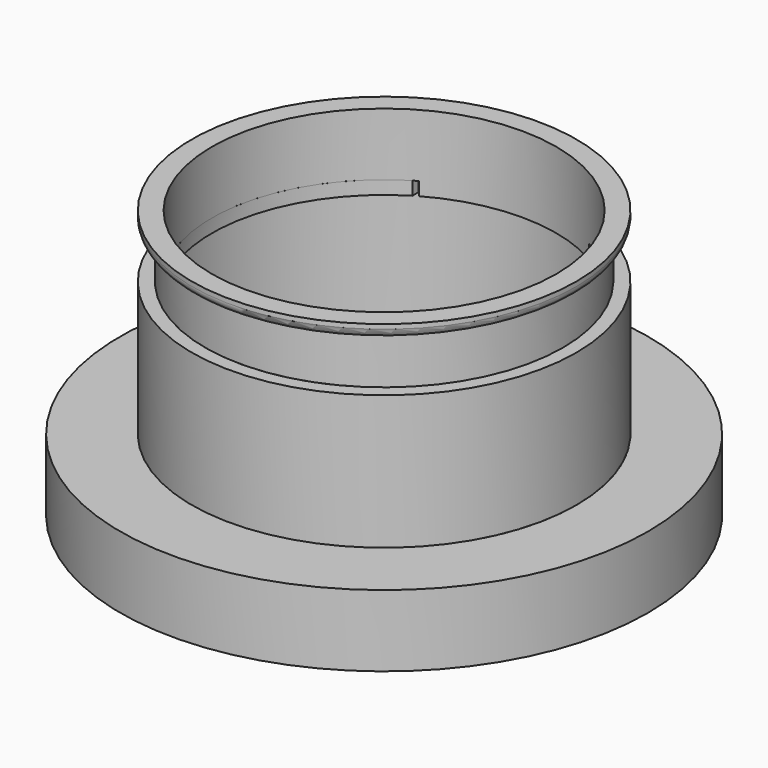
from build123d import *
from build123d import SkipClean  # not in build123d's __all__

# Parameters (mm, degrees)
F1_R      = 29.5
F2_DEPTH  = 8
F0_R      = 28
F3_DEPTH  = 6
F4_R      = 21.5
F5_DEPTH  = 15
F6_R      = 20.75
F7_DEPTH  = 21.5
F8_R      = 20
F9_DEPTH  = 7
F12_DEPTH = 1.5
F14_DEPTH = 2
F15_DEPTH = 1.5
F17_DEPTH = 2
F19_DEPTH = 2
F20_R     = 0.49999
F20_2_R   = 0.49999
F21_R     = 21.5
F22_DEPTH = 1.5
F10_R     = 19.25
F23_DEPTH = 50
F24_R     = 1


# Not quite as in the source:
# - a fillet or chamfer is up to 0.001 mm smaller than in the source, because OpenCascade refuses the exact size
# - a feature of the source that left no trace in its solid (it failed there, or was rolled back) is left out


with BuildPart() as f2:
    # F1 (on Top) → F2 (new body)
    with BuildSketch(Plane.XY):
        Circle(F1_R)
    extrude(amount=F2_DEPTH)

    # F0 (on Top) → F3 (cut)
    with BuildSketch(Plane.XY):
        Circle(F0_R)
    extrude(amount=F3_DEPTH, mode=Mode.SUBTRACT)


with BuildPart() as f5:
    # F4 (on face) → F5 (new body)
    with BuildSketch(Plane.XY.offset(8)):
        Circle(F4_R)
    extrude(amount=F5_DEPTH)


with BuildPart() as f7_tool:
    # F6 (on Top) → F7 (new body)
    with BuildSketch(Plane.XY):
        Circle(F6_R)
    extrude(amount=F7_DEPTH)


with BuildPart() as f2_1:
    add(f2.part, clean=False)

    # F7: cut by f7_tool
    add(f7_tool.part, mode=Mode.SUBTRACT)

    # F11 (on face) → F14 (cut)
    with BuildSketch(Plane(origin=(0, 0, 21.5), x_dir=(1, 0, 0), z_dir=(0, 0, -1))):
        with BuildLine():
            ThreePointArc((10, 17.3205080757), (0, 20), (-10, 17.3205080757))
            Line((-10, 17.3205080757), (-10, -17.3205080757))
            ThreePointArc((-10, -17.3205080757), (0, -20), (10, -17.3205080757))
            Line((10, -17.3205080757), (10, 17.3205080757))
        make_face()
    extrude(amount=F14_DEPTH, mode=Mode.SUBTRACT)

    # F16 (on face) → F17 (cut)
    with BuildSketch(Plane(origin=(0, 0, 6), x_dir=(1, 0, 0), z_dir=(0, 0, -1))):
        with BuildLine():
            Line((-18.1813778356, 10), (-19.0328663107, 10))
            ThreePointArc((-19.0328663107, 10), (-21.5, 0), (-19.0328663107, -10))
            Line((-19.0328663107, -10), (-18.1813778356, -10))
            ThreePointArc((-18.1813778356, -10), (-20.75, 0), (-18.1813778356, 10))
        make_face()
        with BuildLine():
            ThreePointArc((21.5, 0), (20.8741062764, 5.1499210829), (19.0328663107, 10))
            Line((19.0328663107, 10), (18.1813778356, 10))
            ThreePointArc((18.1813778356, 10), (20.0975880405, 5.1623110092), (20.75, 0))
            ThreePointArc((20.75, 0), (20.0975880405, -5.1623110092), (18.1813778356, -10))
            Line((18.1813778356, -10), (19.0328663107, -10))
            ThreePointArc((19.0328663107, -10), (20.8741062764, -5.1499210829), (21.5, 0))
        make_face()
    extrude(amount=-F17_DEPTH, mode=Mode.SUBTRACT)

    # F20 (radius 0.5 in the source; OpenCascade refuses exactly that, so slightly less here)
    f20_edges = [f2_1.edges().sort_by_distance(p)[0] for p in [
        (-28, 0, 0),
        (0, -20.75, 6),
        (0, 20.75, 6),
    ]]
    fillet(f20_edges, radius=F20_R)


with BuildPart() as f5_1:
    add(f5.part, clean=False)

    # F7: cut by f7_tool
    add(f7_tool.part, mode=Mode.SUBTRACT)

    # F11 (on face) → F12 (cut)
    with BuildSketch(Plane(origin=(0, 0, 21.5), x_dir=(1, 0, 0), z_dir=(0, 0, -1))):
        with BuildLine():
            ThreePointArc((10, 17.3205080757), (0, 20), (-10, 17.3205080757))
            Line((-10, 17.3205080757), (-10, -17.3205080757))
            ThreePointArc((-10, -17.3205080757), (0, -20), (10, -17.3205080757))
            Line((10, -17.3205080757), (10, 17.3205080757))
        make_face()
    extrude(amount=-F12_DEPTH, mode=Mode.SUBTRACT)

    # F18 (on face) → F19 (join)
    with BuildSketch(Plane(origin=(0, 0, 8), x_dir=(1, 0, 0), z_dir=(0, 0, -1))):
        with BuildLine():
            Line((-18.4475608144, 9.5), (-19.0082219053, 9.5))
            ThreePointArc((-19.0082219053, 9.5), (-21.25, 0), (-19.0082219053, -9.5))
            Line((-19.0082219053, -9.5), (-18.4475608144, -9.5))
            ThreePointArc((-18.4475608144, -9.5), (-20.75, 0), (-18.4475608144, 9.5))
        make_face()
        with BuildLine():
            ThreePointArc((21.25, 0), (20.6819633435, 4.8804602505), (19.0082219053, 9.5))
            Line((19.0082219053, 9.5), (18.4475608144, 9.5))
            ThreePointArc((18.4475608144, 9.5), (20.1661769666, 4.887515376), (20.75, 0))
            ThreePointArc((20.75, 0), (20.1661769666, -4.887515376), (18.4475608144, -9.5))
            Line((18.4475608144, -9.5), (19.0082219053, -9.5))
            ThreePointArc((19.0082219053, -9.5), (20.6819633435, -4.8804602505), (21.25, 0))
        make_face()
    with SkipClean():  # cleaning this boolean's faces spoils the solid; the shape is the same uncleaned
        extrude(amount=F19_DEPTH)

    # F20#2 (radius 0.5 in the source; OpenCascade refuses exactly that, so slightly less here)
    f20_2_edges = [f5_1.edges().sort_by_distance(p)[0] for p in [
        (20.75, 0, 6),
        (-20.75, 0, 6),
    ]]
    fillet(f20_2_edges, radius=F20_2_R)


with BuildPart() as f9:
    # F8 (on face) → F9 (new body)
    with BuildSketch(Plane.XY.offset(23)):
        Circle(F8_R)
    extrude(amount=F9_DEPTH)

    # F13 (on face) → F15 (join)
    with BuildSketch(Plane(origin=(0, 0, 23), x_dir=(1, 0, 0), z_dir=(0, 0, -1))):
        with BuildLine():
            ThreePointArc((9.5, 17.3150945709), (0, 19.75), (-9.5, 17.3150945709))
            Line((-9.5, 17.3150945709), (-9.5, -17.3150945709))
            ThreePointArc((-9.5, -17.3150945709), (0, -19.75), (9.5, -17.3150945709))
            Line((9.5, -17.3150945709), (9.5, 17.3150945709))
        make_face()
    extrude(amount=F15_DEPTH)

    # F21 (on face) → F22 (join)
    with BuildSketch(Plane.XY.offset(30)):
        Circle(F21_R)
    extrude(amount=-F22_DEPTH)


with BuildPart() as f23_tool:
    # F10 (on Top) → F23 (new body)
    with BuildSketch(Plane.XY):
        Circle(F10_R)
    extrude(amount=F23_DEPTH)


with BuildPart() as f5_2:
    add(f5_1.part, clean=False)

    # F23: cut by f23_tool
    add(f23_tool.part, mode=Mode.SUBTRACT)


with BuildPart() as f9_1:
    add(f9.part, clean=False)

    # F23: cut by f23_tool
    add(f23_tool.part, mode=Mode.SUBTRACT)

    # F24
    f24_edges = [f9_1.edges().sort_by_distance(p)[0] for p in [
        (-21.5, 0, 28.5),
    ]]
    fillet(f24_edges, radius=F24_R)


solid = Compound([f2_1.part, f5_2.part, f9_1.part])
